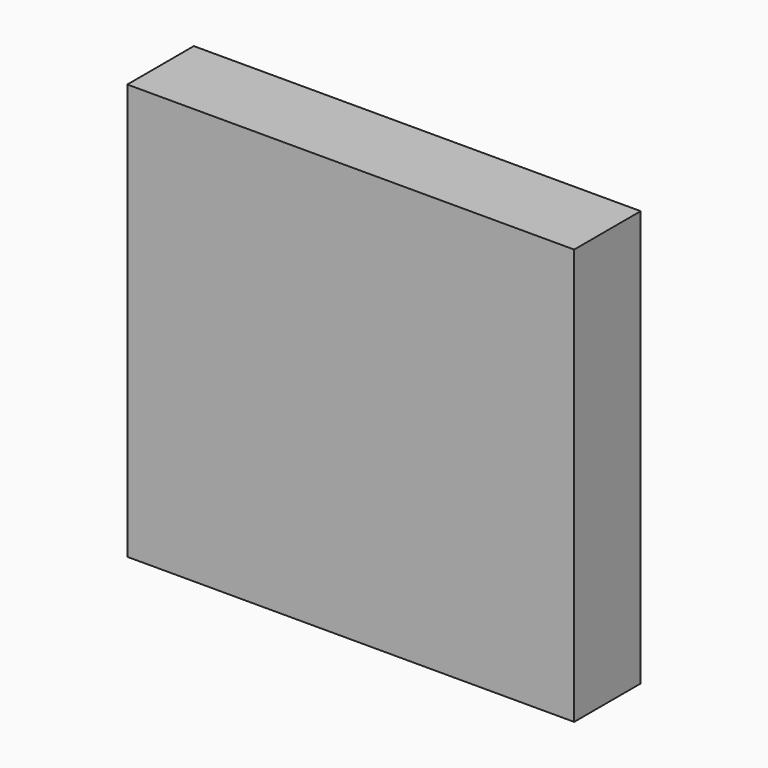
from build123d import *

# Parameters (mm, degrees)
F1_E0_BOTTOM_W = 136.4749222994
F1_E0_BOTTOM_H = 25.4
F2_DEPTH       = 127


with BuildPart() as f2:
    # F1_E0_bottom (on explicit) → F2 (new body)
    with BuildSketch(Plane(origin=(-21.976724267, 0, -37.7777703106), x_dir=(1, 0, 0), z_dir=(0, 0, -1))):
        with Locations((68.2374611497, 12.7)):
            Rectangle(F1_E0_BOTTOM_W, F1_E0_BOTTOM_H)
    extrude(amount=F2_DEPTH)


solid = f2.part
